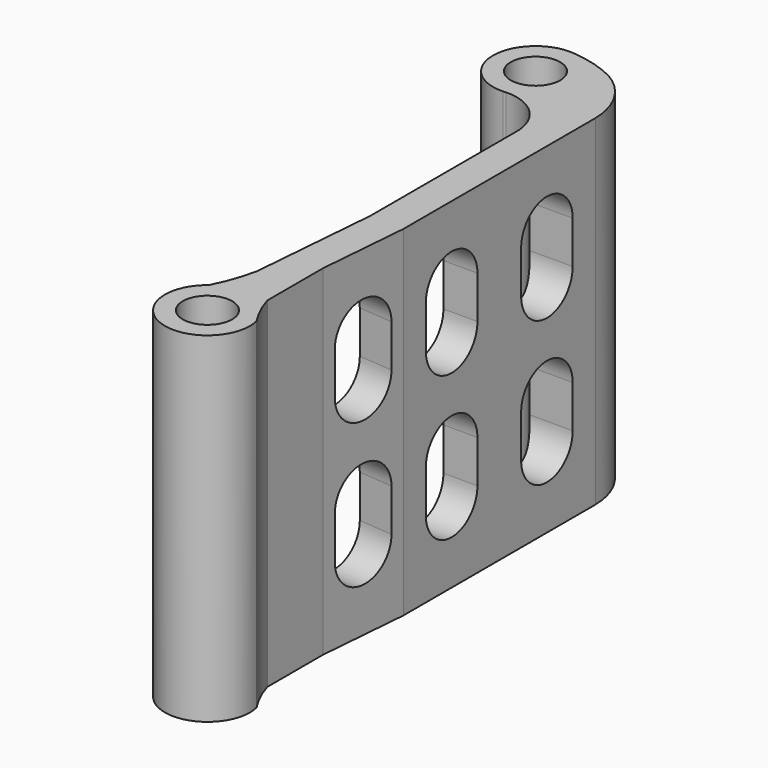
from build123d import *

# Parameters (mm, degrees)
F0_R     = 1.45
F1_DEPTH = 20
F3_DEPTH = 25
F5_DEPTH = 25


# Not quite as in the source:
# - a feature names something its author has since deleted; it is built from what else it names


with BuildPart() as f1:
    # F0 (on Top) → F1 (new body)
    with BuildSketch(Plane.XY):
        with BuildLine():
            Line((5.2166173299, -7.3856279958), (5.6577173299, -2.0351279958))
            Line((5.6577173299, -2.0351279958), (5.6577173299, 12.0690828189))
            ThreePointArc((5.6577173299, 12.0690828189), (5.068252548, 14.1845927754), (3.5162961604, 15.7383889255))
            ThreePointArc((3.5162961604, 15.7383889255), (2.260074285, 16.2332107279), (0.9331621041, 16.4827023722))
            ThreePointArc((0.9331621041, 16.4827023722), (2.4795483886, 15.6499153849), (3.0965173299, 14.0054720042))
            ThreePointArc((3.0965173299, 14.0054720042), (2.4482954337, 12.3259131769), (0.8397830463, 11.5173357959))
            ThreePointArc((0.8397830463, 11.5173357959), (2.7724359809, 10.8070477652), (3.6577173299, 8.9480336756))
            Line((3.6577173299, 8.9480336756), (3.6577173299, -1.9528267058))
            Line((3.6577173299, -1.9528267058), (3.2233793816, -7.2213036786))
            Line((3.2233793816, -7.2213036786), (3.0354523847, -9.5008398307))
            ThreePointArc((3.0354523847, -9.5008398307), (2.6844675314, -10.7628559885), (2.1688231186, -11.9670096287))
            ThreePointArc((2.1688231186, -11.9670096287), (2.8315798002, -16.3061539408), (6.1209868425, -13.3997435963))
            ThreePointArc((6.1209868425, -13.3997435963), (5.5965527788, -12.467225095), (5.2166173299, -11.4670896557))
            Line((5.2166173299, -11.4670896557), (5.2166173299, -7.3856279958))
        make_face()
        with Locations((3.6836173299, -13.9558279958)):
            Circle(F0_R, mode=Mode.SUBTRACT)
        with BuildLine():
            ThreePointArc((0.5965173299, 16.5054720042), (0.7649742372, 16.4960760435), (0.9331621041, 16.4827023722))
            ThreePointArc((0.9331621041, 16.4827023722), (0.7652242949, 16.4997731007), (0.5965173299, 16.5054720042))
        make_face()
        with BuildLine():
            ThreePointArc((3.0965173299, 14.0054720042), (2.4795483886, 15.6499153849), (0.9331621041, 16.4827023722))
            ThreePointArc((0.9331621041, 16.4827023722), (0.7649742372, 16.4960760435), (0.5965173299, 16.5054720042))
            ThreePointArc((0.5965173299, 16.5054720042), (-1.903159389, 13.9652687601), (0.6769134206, 11.5067650449))
            ThreePointArc((0.6769134206, 11.5067650449), (0.7582691412, 11.5132690403), (0.8397830463, 11.5173357959))
            ThreePointArc((0.8397830463, 11.5173357959), (2.4482954337, 12.3259131769), (3.0965173299, 14.0054720042))
        make_face()
        with Locations((0.5965173299, 14.0054720042)):
            Circle(F0_R, mode=Mode.SUBTRACT)
        with BuildLine():
            ThreePointArc((0.6769134206, 11.5067650449), (0.7584345203, 11.5107209498), (0.8397830463, 11.5173357959))
            ThreePointArc((0.8397830463, 11.5173357959), (0.7582691412, 11.5132690403), (0.6769134206, 11.5067650449))
        make_face()
    extrude(amount=F1_DEPTH)

    # F2 (on face) → F3 (cut)
    with BuildSketch(Plane.YZ.offset(5.6577173299)):
        with BuildLine():
            Line((3.4114552828, 13), (3.4114552828, 15.5))
            ThreePointArc((3.4114552828, 15.5), (1.5169774116, 17.3944778712), (-0.3775004597, 15.5))
            Line((-0.3775004597, 15.5), (-0.3775004597, 13))
            ThreePointArc((-0.3775004597, 13), (1.5169774116, 11.1055221288), (3.4114552828, 13))
        make_face()
        with BuildLine():
            Line((6.6224995403, 7), (6.6224995403, 4.5))
            ThreePointArc((6.6224995403, 4.5), (8.5169774116, 2.6055221288), (10.4114552828, 4.5))
            Line((10.4114552828, 4.5), (10.4114552828, 7))
            ThreePointArc((10.4114552828, 7), (8.5169774116, 8.8944778712), (6.6224995403, 7))
        make_face()
        with BuildLine():
            ThreePointArc((10.4114552828, 15.5), (8.5169774116, 17.3944778712), (6.6224995403, 15.5))
            Line((6.6224995403, 15.5), (6.6224995403, 13))
            ThreePointArc((6.6224995403, 13), (8.5169774116, 11.1055221288), (10.4114552828, 13))
            Line((10.4114552828, 13), (10.4114552828, 15.5))
        make_face()
        with BuildLine():
            ThreePointArc((-0.3775004597, 4.5), (1.5169774116, 2.6055221288), (3.4114552828, 4.5))
            Line((3.4114552828, 4.5), (3.4114552828, 7))
            ThreePointArc((3.4114552828, 7), (1.5169774116, 8.8944778712), (-0.3775004597, 7))
            Line((-0.3775004597, 7), (-0.3775004597, 4.5))
        make_face()
    extrude(amount=-F3_DEPTH, mode=Mode.SUBTRACT)

    # F4 (on face) → F5 (cut)
    with BuildSketch(Plane(origin=(5.7861693945, -0.4770169741, 0), x_dir=(0.0821621586, 0.9966189742, 0), z_dir=(0.9966189742, -0.0821621586, 0))):
        with BuildLine():
            ThreePointArc((-2.3532448105, 15.5), (-4.2477226817, 17.3944778712), (-6.142200553, 15.5))
            Line((-6.142200553, 15.5), (-6.142200553, 13))
            ThreePointArc((-6.142200553, 13), (-4.2477226817, 11.1055221288), (-2.3532448105, 13))
            Line((-2.3532448105, 13), (-2.3532448105, 15.5))
        make_face()
        with BuildLine():
            ThreePointArc((-6.142200553, 4.5), (-4.2477226817, 2.6055221288), (-2.3532448105, 4.5))
            Line((-2.3532448105, 4.5), (-2.3532448105, 7))
            ThreePointArc((-2.3532448105, 7), (-4.2477226817, 8.8944778712), (-6.142200553, 7))
            Line((-6.142200553, 7), (-6.142200553, 4.5))
        make_face()
    extrude(amount=-F5_DEPTH, mode=Mode.SUBTRACT)


solid = f1.part
